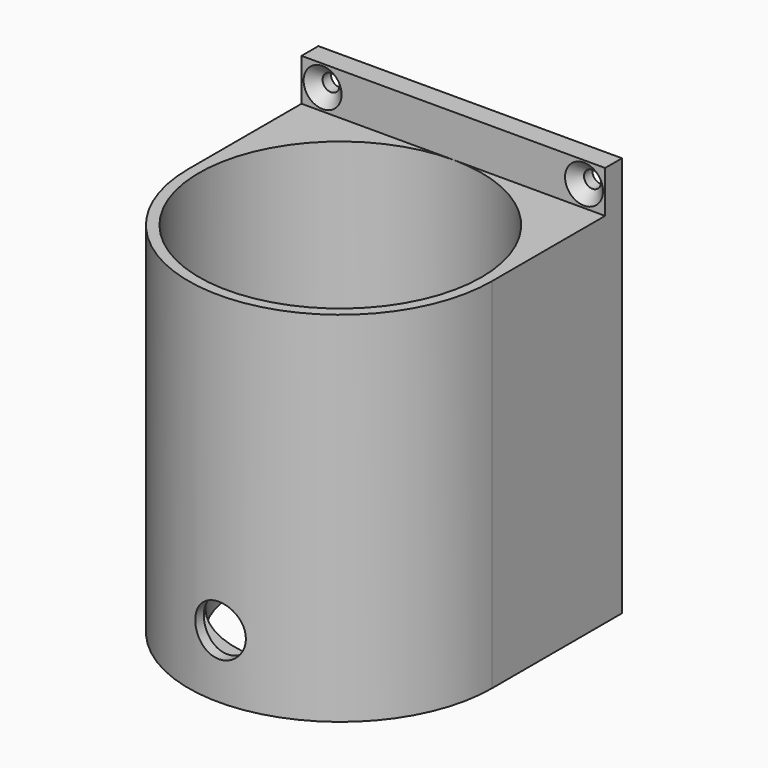
from build123d import *
from build123d import SkipClean  # not in build123d's __all__

# Parameters (mm, degrees)
F1_DEPTH        = 95
F2_W            = 72
F2_H            = 80
F3_DEPTH        = 10
F4_R            = 33.5
F5_DEPTH        = 80
F7_D            = 4
F7_CSINK_D      = 9
F7_CSINK_ANGLE  = 90
F7_COPIES_COUNT = 2
F7_COPIES_PITCH = 81.154174
F8_R            = 25
F9_DEPTH        = 5.001
F11_R           = 6
F12_DEPTH       = 73.5


# Not quite as in the source:
# - a feature of the source that left no trace in its solid (it failed there, or was rolled back) is left out
# - a pattern or mirror of a feature is missing from the dataset's text; its kind, count and spacing are read off the source's solid


with BuildPart() as f1:
    # F0 (on Top) → F1 (new body)
    with BuildSketch(Plane.XY):
        with BuildLine():
            Line((36, 38.5), (-36, 38.5))
            Line((-36, 38.5), (-36, 0))
            ThreePointArc((-36, 0), (0, -36), (36, 0))
            Line((36, 0), (36, 38.5))
        make_face()
    extrude(amount=F1_DEPTH)

    # F2 (on face) → F3 (cut)
    with BuildSketch(Plane.XY.offset(95)):
        with Locations((0, -6.5)):
            Rectangle(F2_W, F2_H)
    extrude(amount=-F3_DEPTH, mode=Mode.SUBTRACT)

    # F4 (on face) → F5 (cut)
    with BuildSketch(Plane.XY.offset(85)):
        Circle(F4_R)
    extrude(amount=-F5_DEPTH, mode=Mode.SUBTRACT)

    # F7 (through all)
    with Locations(Plane.XZ.offset(-33.5)):
        with Locations((-31, 90), (31, 90)):
            f7 = CounterSinkHole(F7_D / 2, F7_CSINK_D / 2, counter_sink_angle=F7_CSINK_ANGLE)

    # F7_copies: F7 ×2
    with Locations(*[Vector(-0.3819889769, 0, -0.9241668797) * (i * F7_COPIES_PITCH) for i in range(1, F7_COPIES_COUNT)]):
        add(f7, clean=False, mode=Mode.SUBTRACT)

    # F8 (on face) → F9 (cut, through all)
    with BuildSketch(Plane.XY.offset(5)):
        Circle(F8_R)
    extrude(amount=-F9_DEPTH, mode=Mode.SUBTRACT)

    # F11 (on offset) → F12 (cut)
    with BuildSketch(Plane.XZ.offset(40)):
        with Locations((0, 15)):
            Circle(F11_R)
    with SkipClean():  # cleaning this boolean's faces spoils the solid; the shape is the same uncleaned
        extrude(amount=-F12_DEPTH, mode=Mode.SUBTRACT)


solid = f1.part
